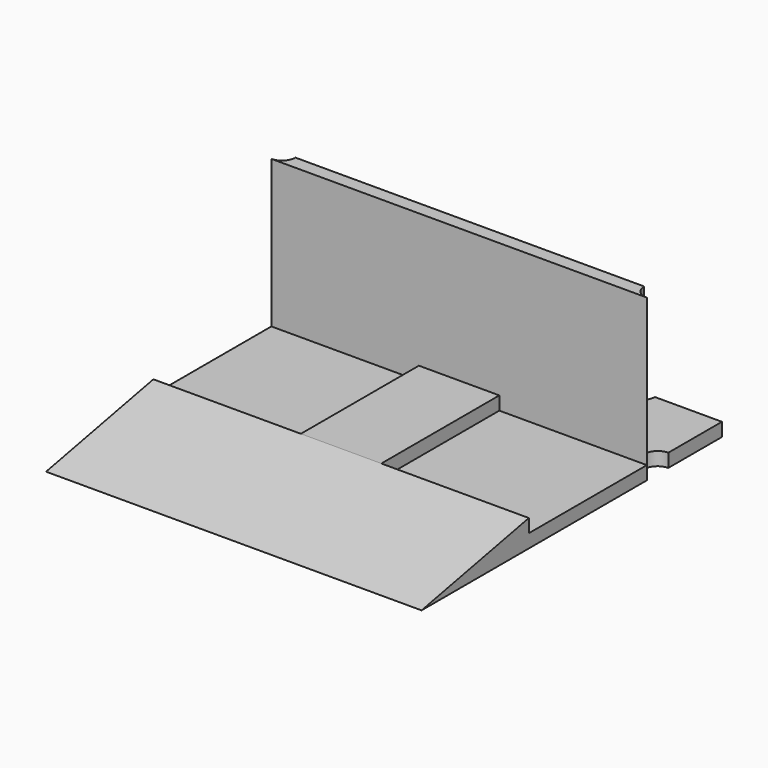
from build123d import *

# Parameters (mm, degrees)
F0_W     = 40.2394990027
F0_H     = 20
F0_W_2   = 55
F0_H_2   = 55
F1_DEPTH = 5
F0_W_3   = 30
F2_DEPTH = 10
F4_DEPTH = 141
F5_DEPTH = 60


# Not quite as in the source:
# - a feature names something its author has since deleted; it is built from what else it names


with BuildPart() as f1:
    # F0 (on Top) → F1 (new body)
    with BuildSketch(Plane.XY):
        with BuildLine():
            Line((-40.5921050906, 26.1479860185), (-65.5921050906, 26.1479860185))
            ThreePointArc((-65.5921050906, 26.1479860185), (-67.0565711847, 22.6124521126), (-70.5921050906, 21.1479860185))
            Line((-70.5921050906, 21.1479860185), (-15.5921050906, 21.1479860185))
            Line((-15.5921050906, 21.1479860185), (14.4078949094, 21.1479860185))
            Line((14.4078949094, 21.1479860185), (69.4078949094, 21.1479860185))
            ThreePointArc((69.4078949094, 21.1479860185), (65.8723610034, 22.6124521126), (64.4078949094, 26.1479860185))
            Line((64.4078949094, 26.1479860185), (39.4078949094, 26.1479860185))
            Line((39.4078949094, 26.1479860185), (-40.5921050906, 26.1479860185))
        make_face()
        with BuildLine():
            Line((-45.5921050906, 56.1479860185), (-70.5921050906, 56.1479860185))
            Line((-70.5921050906, 56.1479860185), (-70.5921050906, 31.1479860185))
            ThreePointArc((-70.5921050906, 31.1479860185), (-67.0565711847, 29.6835199245), (-65.5921050906, 26.1479860185))
            Line((-65.5921050906, 26.1479860185), (-40.5921050906, 26.1479860185))
            Line((-40.5921050906, 26.1479860185), (-40.5921050906, 51.1479860185))
            ThreePointArc((-40.5921050906, 51.1479860185), (-44.1276389966, 52.6124521126), (-45.5921050906, 56.1479860185))
        make_face()
        with Locations((-0.5921050906, 46.1479860185)):
            Rectangle(F0_W, F0_H)
        with BuildLine():
            Line((39.4078949094, 51.1479860185), (39.4078949094, 26.1479860185))
            Line((39.4078949094, 26.1479860185), (64.4078949094, 26.1479860185))
            ThreePointArc((64.4078949094, 26.1479860185), (65.8723610034, 29.6835199245), (69.4078949094, 31.1479860185))
            Line((69.4078949094, 31.1479860185), (69.4078949094, 56.1479860185))
            Line((69.4078949094, 56.1479860185), (44.4078949094, 56.1479860185))
            ThreePointArc((44.4078949094, 56.1479860185), (42.9434288153, 52.6124521126), (39.4078949094, 51.1479860185))
        make_face()
        with BuildLine():
            ThreePointArc((-35.5921050906, 56.1479860185), (-37.0565711847, 52.6124521126), (-40.5921050906, 51.1479860185))
            Line((-40.5921050906, 51.1479860185), (-40.5921050906, 26.1479860185))
            Line((-40.5921050906, 26.1479860185), (39.4078949094, 26.1479860185))
            Line((39.4078949094, 26.1479860185), (39.4078949094, 51.1479860185))
            ThreePointArc((39.4078949094, 51.1479860185), (35.8723610034, 52.6124521126), (34.4078949094, 56.1479860185))
            Line((34.4078949094, 56.1479860185), (22.5276444107, 56.1479860185))
            Line((22.5276444107, 56.1479860185), (22.5276444107, 36.1479860185))
            Line((22.5276444107, 36.1479860185), (19.5276444107, 36.1479860185))
            Line((19.5276444107, 36.1479860185), (-20.711854592, 36.1479860185))
            Line((-20.711854592, 36.1479860185), (-23.711854592, 36.1479860185))
            Line((-23.711854592, 36.1479860185), (-23.711854592, 56.1479860185))
            Line((-23.711854592, 56.1479860185), (-35.5921050906, 56.1479860185))
        make_face()
        with Locations((-43.0921050906, -6.3520139815)):
            Rectangle(F0_W_2, F0_H_2)
        with Locations((41.9078949094, -6.3520139815)):
            Rectangle(F0_W_2, F0_H_2)
    extrude(amount=F1_DEPTH)

    # F0 (on Top) → F2 (join)
    with BuildSketch(Plane.XY):
        with Locations((-0.5921050906, -6.3520139815)):
            Rectangle(F0_W_3, F0_H_2)
        Polygon((-15.5921050906, -33.8520139815), (-70.5921050906, -33.8520139815), (-70.5921050906, -83.8520139815), (69.4078949094, -83.8520139815), (69.4078949094, -33.8520139815), (14.4078949094, -33.8520139815), align=None)
    extrude(amount=F2_DEPTH)

    # F3 (on face) → F4 (cut)
    with BuildSketch(Plane(origin=(-70.5921050906, 0, 0), x_dir=(0, -1, 0), z_dir=(-1, 0, 0))):
        Polygon((83.8520139815, 10), (33.8520139815, 10), (83.8520139815, 0), align=None)
    extrude(amount=-F4_DEPTH, mode=Mode.SUBTRACT)

    # F0 (on Top) → F5 (join)
    with BuildSketch(Plane.XY):
        with BuildLine():
            Line((-40.5921050906, 26.1479860185), (-65.5921050906, 26.1479860185))
            ThreePointArc((-65.5921050906, 26.1479860185), (-67.0565711847, 22.6124521126), (-70.5921050906, 21.1479860185))
            Line((-70.5921050906, 21.1479860185), (-15.5921050906, 21.1479860185))
            Line((-15.5921050906, 21.1479860185), (14.4078949094, 21.1479860185))
            Line((14.4078949094, 21.1479860185), (69.4078949094, 21.1479860185))
            ThreePointArc((69.4078949094, 21.1479860185), (65.8723610034, 22.6124521126), (64.4078949094, 26.1479860185))
            Line((64.4078949094, 26.1479860185), (39.4078949094, 26.1479860185))
            Line((39.4078949094, 26.1479860185), (-40.5921050906, 26.1479860185))
        make_face()
    extrude(amount=F5_DEPTH)


solid = f1.part
